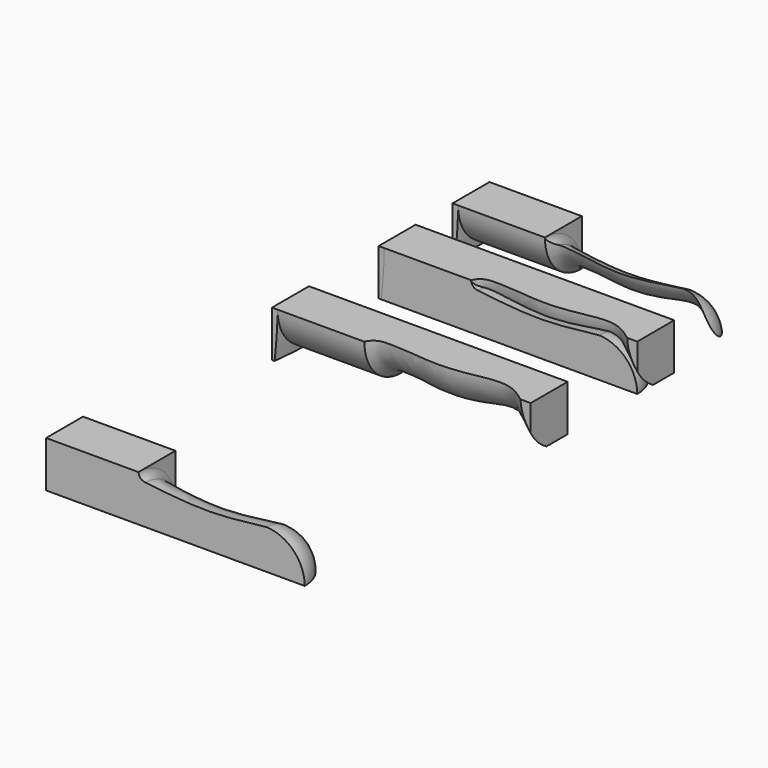
from build123d import *

# Parameters (mm, degrees)
F0_W     = 50
F0_H     = 50
F1_DEPTH = 280
F2_W     = 180
F2_H     = 24.827849865
F3_ANGLE = 90
F4_W     = 50
F4_H     = 50
F5_DEPTH = 280
F7_ANGLE = 90


# Not quite as in the source:
# - a feature names something its author has since deleted; it is built from what else it names


with BuildPart() as f1:
    # F0 (on Right) → F1 (new body)
    with BuildSketch(Plane.YZ):
        with Locations((25, 25)):
            Rectangle(F0_W, F0_H)
    extrude(amount=F1_DEPTH)

    # F2 (on face) → F3 (revolve, cut)
    with BuildSketch(Plane.XZ):
        with BuildLine():
            ThreePointArc((238.8043701649, 42.6135770977), (268.0173314079, 29.6352698257), (280, 0))
            Line((280, 0), (280, 50))
            Line((280, 50), (100, 50))
            ThreePointArc((100, 50), (102.3815317412, 44.7572932157), (107.7258884907, 42.6135770977))
            add(Edge.make_bspline(
                [(238.8043701649, 42.6135770977), (216.8314378852, 40.0097605898), (172.9862871231, 34.8140622694), (129.446016876, 40.01772315), (107.7258884907, 42.6135770977)],
                knots=[0, 0, 0, 0, 0.5011485169, 1, 1, 1, 1], degree=3))
        make_face()
        with Locations((190, 62.4139249325)):
            Rectangle(F2_W, F2_H)
    revolve(axis=Axis((140, 0, 0), (-1, 0, 0)), revolution_arc=F3_ANGLE, mode=Mode.SUBTRACT)


with BuildPart() as f5:
    # F4 (on Right) → F5 (new body)
    with BuildSketch(Plane.YZ):
        with Locations((330.7065606117, 25)):
            Rectangle(F4_W, F4_H)
    extrude(amount=F5_DEPTH)

    # F6 (on face) → F7 (revolve, cut)
    with BuildSketch(Plane(origin=(0, 355.7065606117, 0), x_dir=(-1, 0, 0), z_dir=(0, 1, 0))):
        with BuildLine():
            add(Edge.make_bspline(
                [(-269.1363870583, 0), (-262.8963183755, 4.6236035117), (-244.5435058692, 17.7466423376), (-208.881742022, 9.2386826676), (-174.0217149646, 4.8240239294), (-139.8010132048, 9.3863383487), (-121.0962155366, 9.9511328259), (-104.7735759931, 10.0222443244), (-100, 0)],
                knots=[0.0697887667, 0.0697887667, 0.0697887667, 0.0697887667, 0.1823413245, 0.3705605147, 0.5520509525, 0.7252963367, 0.8569887429, 1, 1, 1, 1], degree=3))
            Line((-269.1363870583, 0), (-100, 0))
        make_face()
        with BuildLine():
            add(Edge.make_bspline(
                [(-280, -7.5857136399), (-276.6333947385, -5.6233561243), (-273.0055723164, -2.8668880834), (-269.1363870583, 0)],
                knots=[0, 0, 0, 0, 0.0697887667, 0.0697887667, 0.0697887667, 0.0697887667], degree=3))
            Line((-280, -7.5857136399), (-280, -39.3132679164))
            Line((-280, -39.3132679164), (-100.7019568713, -39.3132679164))
            Line((-100.7019568713, -39.3132679164), (-90.5555039644, 0))
            Line((-90.5555039644, 0), (-100, 0))
            Line((-100, 0), (-269.1363870583, 0))
        make_face()
        Polygon((-90.5555039644, 0), (-100.7019568713, -39.3132679164), (0, -39.3132679164), (-5.9527931735, 0), (-10.410037823, 0), align=None)
    revolve(axis=Axis((140, 355.7065606117, 50), (-1, 0, 0)), revolution_arc=F7_ANGLE, mode=Mode.SUBTRACT)


with BuildPart() as f8_1:
    # F8: copy of F1
    add(f1.part.moved(Location((0, 400, 0))))


with BuildPart() as f9_1:
    # F9: copy of F5
    add(f5.part.moved(Location((0, 94.2934393883, 0))))


with BuildPart() as f8_1_1:
    # F10: moved
    add(f8_1.part.moved(Location((0, 50, 0))))


with BuildPart() as f9_1_1:
    # F10: moved
    add(f9_1.part.moved(Location((0, 50, 0))))


with BuildPart() as f11_1:
    # F11: copy of F8_1
    add(f8_1_1.part.moved(Location((0, 100, 0))))


with BuildPart() as f11_2:
    # F11: copy of F9_1
    add(f9_1_1.part.moved(Location((0, 100, 0))))

    # F12: intersect F11_1
    add(f11_1.part, mode=Mode.INTERSECT)


solid = Compound([f1.part, f5.part, f8_1_1.part, f9_1_1.part, f11_2.part])
